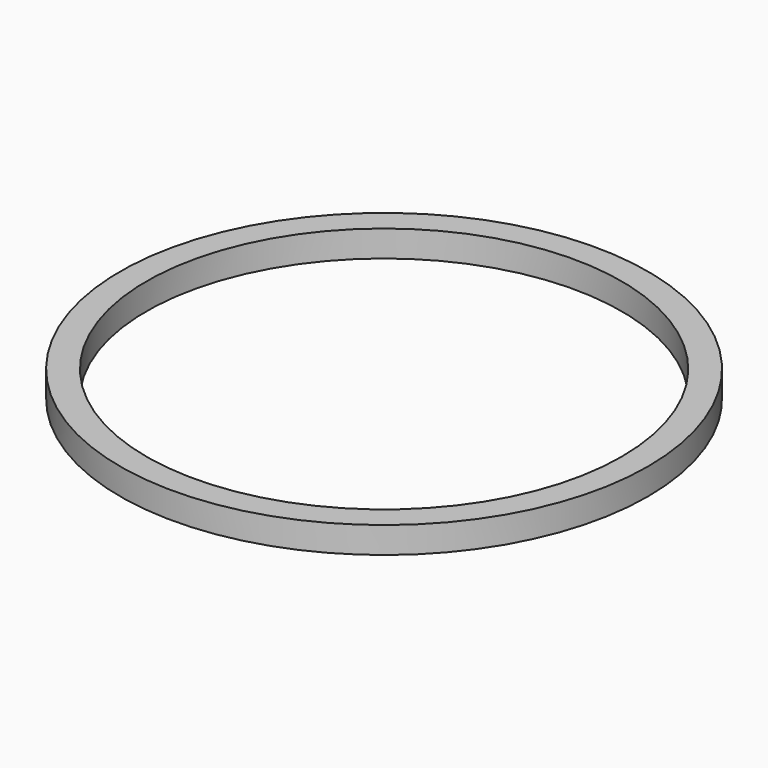
from build123d import *

# Parameters (mm, degrees)
F0_R     = 100
F0_R_2   = 90
F1_DEPTH = 10


# Not quite as in the source:
# - a feature names something its author has since deleted; it is built from what else it names


with BuildPart() as f1:
    # F0 (on Top) → F1 (new body)
    with BuildSketch(Plane.XY):
        Circle(F0_R)
        Circle(F0_R_2, mode=Mode.SUBTRACT)
    extrude(amount=F1_DEPTH)


solid = f1.part
